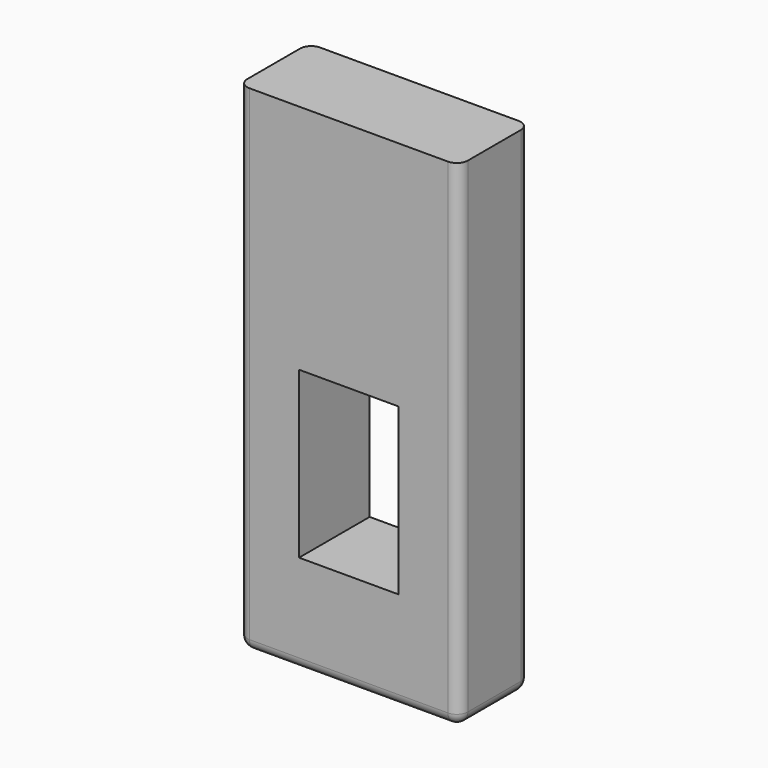
from build123d import *

# Parameters (mm, degrees)
F0_W         = 2
F0_H         = 4.5
F1_DEPTH     = 0.8
F3_DEPTH     = 25.4
F4_R         = 0.1
F5_T1_DEPTH  = 0.6
F5_S5_W      = 0.1
F5_S5_H      = 0.1
F5_T6_DEPTH  = 0.1
F5_S11_W     = 0.1
F5_S11_H     = 0.1
F5_T12_DEPTH = 0.1
F5_S17_W     = 0.1
F5_S17_H     = 0.1
F5_T18_DEPTH = 0.1
F5_S23_W     = 0.1
F5_S23_H     = 0.1
F5_T24_DEPTH = 0.1


# Not quite as in the source:
# - a fillet or chamfer that OpenCascade refuses, or shapes differently, is made with other operations: its cross-section is extruded or revolved along the edge and cut away or added


with BuildPart() as f1:
    # F0 (on Front) → F1 (new body)
    with BuildSketch(Plane.XZ):
        with Locations((1, 2.25)):
            Rectangle(F0_W, F0_H)
    extrude(amount=F1_DEPTH)

    # F2 (on face) → F3 (cut)
    with BuildSketch(Plane.XZ.offset(0.8)):
        Polygon((0.55, 0.9), (1, 0.9), (1.45, 0.9), (1.45, 2.4), (0.55, 2.4), align=None)
    extrude(amount=-F3_DEPTH, mode=Mode.SUBTRACT)

    # F4
    f4_edges = [f1.edges().sort_by_distance(p)[0] for p in [
        (2, -0.8, 2.25),
        (1, -0.8, 0),
        (0, -0.8, 2.25),
        (2, 0, 2.25),
        (1, 0, 0),
        (0, 0, 2.25),
    ]]
    fillet(f4_edges, radius=F4_R)

    # F5: fillet of radius 0.1 on 2 edges, made by hand

    # F5_s2 → F5_t1 (cut)
    with BuildSketch(Plane.XZ.offset(0.1)):
        with BuildLine():
            ThreePointArc((0, 0.1), (0.0292893219, 0.0292893219), (0.1, 0))
            Line((0.1, 0), (0, 0))
            Line((0, 0), (0, 0.1))
        make_face()
        with BuildLine():
            ThreePointArc((1.9, 0), (1.9707106781, 0.0292893219), (2, 0.1))
            Line((2, 0.1), (2, 0))
            Line((2, 0), (1.9, 0))
        make_face()
    extrude(amount=F5_T1_DEPTH, mode=Mode.SUBTRACT)


with BuildPart() as f5_tool4:
    # F5_s5 → F5_t6 (new body)
    with BuildSketch(Plane.XY.offset(0.1)):
        with Locations((1.95, -0.05)):
            Rectangle(F5_S5_W, F5_S5_H)
    extrude(amount=-F5_T6_DEPTH)

    # F5_s7 → F5_t8 (revolve, cut)
    with BuildSketch(Plane(origin=(1.9, -0.1, 0.1), x_dir=(-0.7071067812, -0.7071067812, 0), z_dir=(0.7071067812, -0.7071067812, 0))):
        with BuildLine():
            ThreePointArc((0, -0.1), (0.1, 0), (0, 0.1))
            Line((0, 0.1), (0, -0.1))
        make_face()
    revolve(axis=Axis((1.9, -0.1, 0.1), (0, 0, -1)), mode=Mode.SUBTRACT)


with BuildPart() as f1_1:
    add(f1.part)

    # F5_t3: cut F5_tool4
    add(f5_tool4.part, mode=Mode.SUBTRACT)


with BuildPart() as f5_tool10:
    # F5_s11 → F5_t12 (new body)
    with BuildSketch(Plane.XY.offset(0.1)):
        with Locations((1.95, -0.75)):
            Rectangle(F5_S11_W, F5_S11_H)
    extrude(amount=-F5_T12_DEPTH)

    # F5_s13 → F5_t14 (revolve, cut)
    with BuildSketch(Plane(origin=(1.9, -0.7, 0.1), x_dir=(-0.7071067812, 0.7071067812, 0), z_dir=(-0.7071067812, -0.7071067812, 0))):
        with BuildLine():
            ThreePointArc((0, -0.1), (0.1, 0), (0, 0.1))
            Line((0, 0.1), (0, -0.1))
        make_face()
    revolve(axis=Axis((1.9, -0.7, 0.1), (0, 0, -1)), mode=Mode.SUBTRACT)


with BuildPart() as f1_2:
    add(f1_1.part)

    # F5_t9: cut F5_tool10
    add(f5_tool10.part, mode=Mode.SUBTRACT)


with BuildPart() as f5_tool16:
    # F5_s17 → F5_t18 (new body)
    with BuildSketch(Plane.YZ.offset(0.1)):
        with Locations((-0.05, 0.05)):
            Rectangle(F5_S17_W, F5_S17_H)
    extrude(amount=-F5_T18_DEPTH)

    # F5_s19 → F5_t20 (revolve, cut)
    with BuildSketch(Plane(origin=(0.1, -0.1, 0.1), x_dir=(0, -0.7071067812, 0.7071067812), z_dir=(0, -0.7071067812, -0.7071067812))):
        with BuildLine():
            ThreePointArc((0, -0.1), (0.1, 0), (0, 0.1))
            Line((0, 0.1), (0, -0.1))
        make_face()
    revolve(axis=Axis((0.1, -0.1, 0.1), (-1, 0, 0)), mode=Mode.SUBTRACT)


with BuildPart() as f1_3:
    add(f1_2.part)

    # F5_t15: cut F5_tool16
    add(f5_tool16.part, mode=Mode.SUBTRACT)


with BuildPart() as f5_tool22:
    # F5_s23 → F5_t24 (new body)
    with BuildSketch(Plane.YZ.offset(0.1)):
        with Locations((-0.75, 0.05)):
            Rectangle(F5_S23_W, F5_S23_H)
    extrude(amount=-F5_T24_DEPTH)

    # F5_s25 → F5_t26 (revolve, cut)
    with BuildSketch(Plane(origin=(0.1, -0.7, 0.1), x_dir=(0, 0.7071067812, 0.7071067812), z_dir=(0, -0.7071067812, 0.7071067812))):
        with BuildLine():
            ThreePointArc((0, -0.1), (0.1, 0), (0, 0.1))
            Line((0, 0.1), (0, -0.1))
        make_face()
    revolve(axis=Axis((0.1, -0.7, 0.1), (-1, 0, 0)), mode=Mode.SUBTRACT)


with BuildPart() as f1_4:
    add(f1_3.part)

    # F5_t21: cut F5_tool22
    add(f5_tool22.part, mode=Mode.SUBTRACT)


solid = f1_4.part
